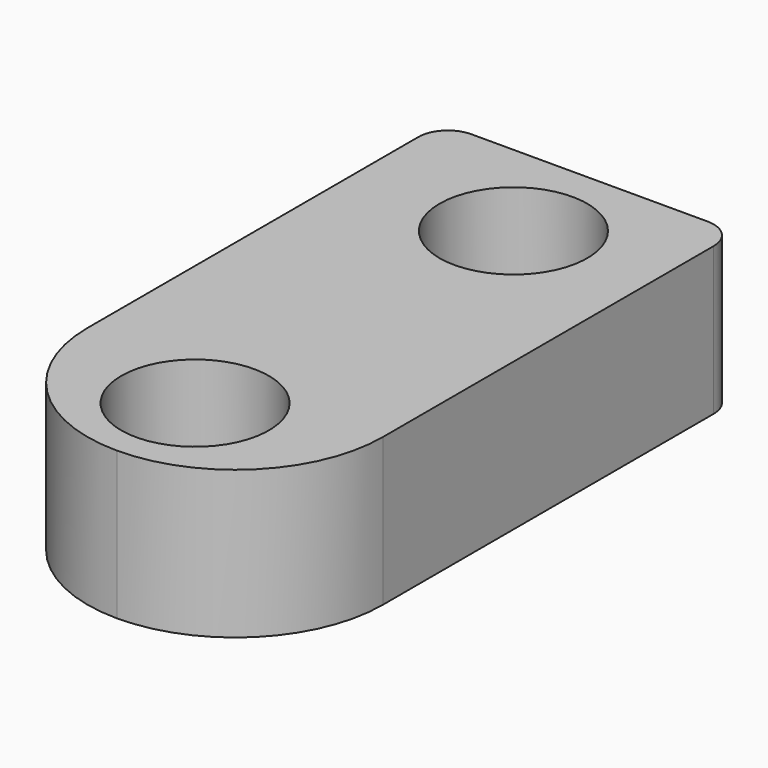
from build123d import *

# Parameters (mm, degrees)
F0_W     = 50.8
F0_H     = 101.6
F1_DEPTH = 25.4
F2_R     = 12.7
F3_DEPTH = 131
F4_D     = 25.4
F6_D     = 25.4
F7_R     = 25.39999
F8_R     = 5.08


# Not quite as in the source:
# - a fillet or chamfer is up to 0.001 mm smaller than in the source, because OpenCascade refuses the exact size
# - an extrude ends at something that could not be found from the text; its depth is read off the source's solid


with BuildPart() as f1:
    # F0 (on Top) → F1 (new body)
    with BuildSketch(Plane.XY):
        with Locations((5.1918309937, -2.1536122621)):
            Rectangle(F0_W, F0_H)
    extrude(amount=F1_DEPTH)

    # F2 (on Top) → F3 (cut, through all)
    with BuildSketch(Plane.XY):
        with Locations((4.7334181145, -35.6077803201)):
            Circle(F2_R)
    extrude(amount=-F3_DEPTH, mode=Mode.SUBTRACT)

    # F4 (through all)
    with Locations(Plane(origin=(0, 0, 0), x_dir=(1, 0, 0), z_dir=(0, 0, -1))):
        with Locations((4.7334181145, 35.6077803201)):
            Hole(F4_D / 2)

    # F6 (through all)
    with Locations(Plane(origin=(0, 0, 0), x_dir=(1, 0, 0), z_dir=(0, 0, -1))):
        with Locations((6.8339584395, -30.2138105035)):
            Hole(F6_D / 2)

    # F7 (radius 25.4 in the source; OpenCascade refuses exactly that, so slightly less here)
    f7_edges = [f1.edges().sort_by_distance(p)[0] for p in [
        (-20.208169, -52.953612, 12.7),
        (30.591831, -52.953612, 12.7),
    ]]
    fillet(f7_edges, radius=F7_R)

    # F8
    f8_edges = [f1.edges().sort_by_distance(p)[0] for p in [
        (-20.208169, 48.646388, 12.7),
        (30.591831, 48.646388, 12.7),
    ]]
    fillet(f8_edges, radius=F8_R)


solid = f1.part
